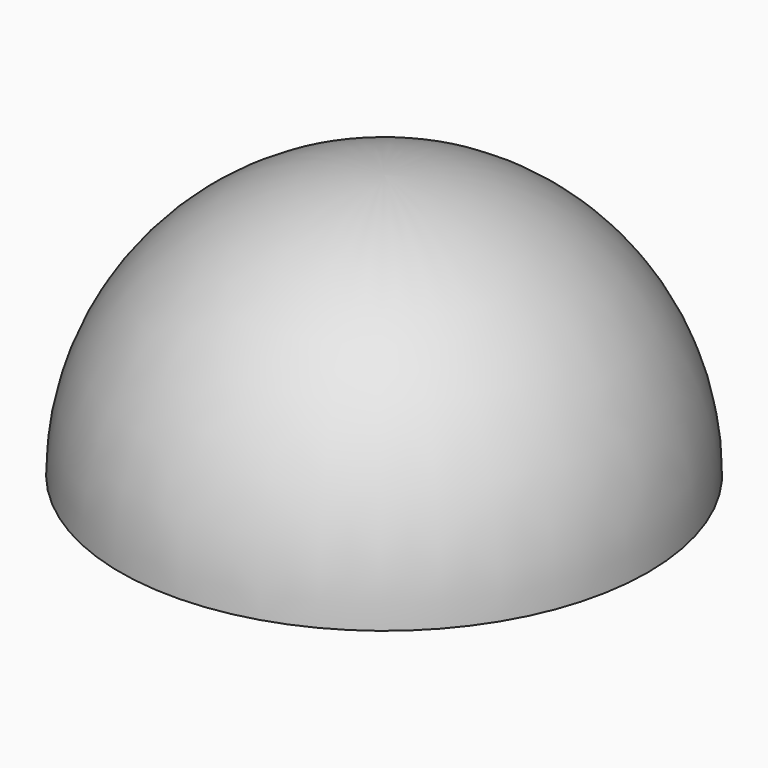
from build123d import *

# Parameters (mm, degrees)
F0_R     = 63.5
F1_DEPTH = 63.5
F2_R     = 63.49999


# Not quite as in the source:
# - a fillet or chamfer is up to 0.001 mm smaller than in the source, because OpenCascade refuses the exact size


with BuildPart() as f1:
    # F0 (on Top) → F1 (new body)
    with BuildSketch(Plane.XY):
        Circle(F0_R)
    extrude(amount=F1_DEPTH)

    # F2 (radius 63.5 in the source; OpenCascade refuses exactly that, so slightly less here)
    f2_edges = [f1.edges().sort_by_distance(p)[0] for p in [
        (-63.5, 0, 63.5),
    ]]
    fillet(f2_edges, radius=F2_R)


solid = f1.part
